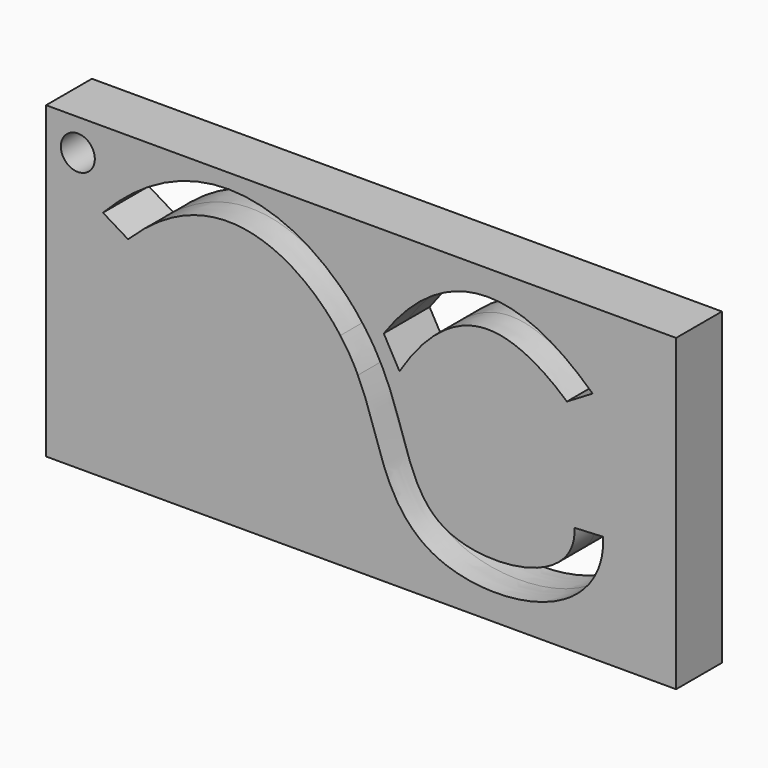
from build123d import *

# Parameters (mm, degrees)
F0_R     = 1.4820473609
F1_DEPTH = 2.5


# Not quite as in the source:
# - ends of sketch curves that miss each other by under 0.0002 mm in the source are joined
# - the dataset's text gives a spline's control points without its knots; the knots are read off the source's solid


with BuildPart() as f1:
    # F0 (on Front) → F1 (new body, symmetric)
    with BuildSketch(Plane.XZ):
        Polygon((0, 8), (0, 35), (-13.424108796, 35), (-19.3373572554, 35), (-55, 35), (-55, 10.4823449254), (-55, 8), align=None)
        with BuildLine():
            add(Edge.make_bspline(
                [(-50.0350917202, 28.3529292792), (-41.4125684769, 37.3503428815), (-32.6083595452, 33.5266259227), (-27.9510231414, 27.9673930825)],
                knots=[0, 0, 0, 0, 0.3600130252, 0.3600130252, 0.3600130252, 0.3600130252], degree=3))
            add(Edge.make_bspline(
                [(-27.9510231414, 27.9673930825), (-27.3487030898, 27.2484333336), (-26.8157416051, 26.5004461928), (-26.3615016308, 25.7474105413)],
                knots=[0.3600130252, 0.3600130252, 0.3600130252, 0.3600130252, 0.4065724843, 0.4065724843, 0.4065724843, 0.4065724843], degree=3))
            add(Edge.make_bspline(
                [(-26.3615016308, 25.7474105413), (-23.3397086824, 20.7379046624), (-24.2248666361, 10.7119674387), (-8.6427712057, 12.8800264919), (-8.8683726817, 17.5248406146)],
                knots=[0.4065724843, 0.4065724843, 0.4065724843, 0.4065724843, 0.7163053419, 1, 1, 1, 1], degree=3))
            Line((-8.8683726817, 17.5248406146), (-6.3713163551, 17.6461241747))
            add(Edge.make_bspline(
                [(-27.7799857666, 23.1064623069), (-27.5788263546, 22.6828182601), (-27.2052833118, 21.8051538248), (-26.5538623577, 19.9878085153), (-25.9771348931, 18.1048414361), (-25.261157142, 16.2105369006), (-24.5732041008, 14.7953607109), (-23.6380951501, 13.4207286348), (-22.5790746848, 12.3877665289), (-21.564555015, 11.6972592795), (-20.7224373548, 11.2571965743), (-19.8357740563, 10.9114121519), (-18.6155851221, 10.5608139887), (-17.024910383, 10.3056128104), (-15.0584946055, 10.2646454513), (-13.0865401909, 10.492714956), (-11.1638473783, 11.0168183507), (-9.6484283114, 11.7525836632), (-8.5378543638, 12.580223758), (-7.781569025, 13.3385124482), (-7.1393061965, 14.2447169704), (-6.6593512732, 15.2903158401), (-6.3849771302, 16.4401002198), (-6.3517175883, 17.2426133896), (-6.3713163551, 17.6461241747)],
                knots=[0.4388333181, 0.4388333181, 0.4388333181, 0.4388333181, 0.46875, 0.5, 0.5625, 0.59375, 0.625, 0.65625, 0.6875, 0.703125, 0.71875, 0.734375, 0.75, 0.78125, 0.8125, 0.84375, 0.875, 0.90625, 0.921875, 0.9375, 0.953125, 0.96875, 0.984375, 1, 1, 1, 1], degree=3))
            add(Edge.make_bspline(
                [(-29.3100691332, 25.6568229932), (-29.175893814, 25.4766680673), (-28.8945520273, 25.081058775), (-28.5026126507, 24.4697850699), (-28.1349969346, 23.8229909625), (-27.9034448496, 23.3653444059), (-27.7889509819, 23.1253431538), (-27.7799857666, 23.1064623069)],
                knots=[0.3774181382, 0.3774181382, 0.3774181382, 0.3774181382, 0.390625, 0.40625, 0.421875, 0.4375, 0.4388333181, 0.4388333181, 0.4388333181, 0.4388333181], degree=3))
            add(Edge.make_bspline(
                [(-47.8384598127, 27.0220131494), (-46.6238688702, 28.2285190868), (-44.7876932656, 29.6157244059), (-42.4668675866, 30.6846781436), (-40.7284615762, 31.1431332011), (-39.0640314859, 31.276428493), (-37.4540401325, 31.1251354681), (-35.8908216692, 30.7151649499), (-33.8798974431, 29.854230091), (-32.0180305429, 28.5725811639), (-30.4090118206, 27.0178615308), (-29.6791632781, 26.1485815571), (-29.3346362458, 25.6898088386), (-29.3100691332, 25.6568229932)],
                knots=[0.0060505396, 0.0060505396, 0.0060505396, 0.0060505396, 0.0625, 0.09375, 0.125, 0.15625, 0.1875, 0.21875, 0.25, 0.3125, 0.34375, 0.375, 0.3774181382, 0.3774181382, 0.3774181382, 0.3774181382], degree=3))
            Line((-47.8384598127, 27.0220131494), (-50.0350917202, 28.3529292792))
        make_face(mode=Mode.SUBTRACT)
        with Locations((-52.2252842784, 32.250855118)):
            Circle(F0_R, mode=Mode.SUBTRACT)
        with BuildLine():
            Line((-24.1447698904, 24.5811181712), (-25.5211698706, 27.0438124237))
            add(Edge.make_bspline(
                [(-25.5211698706, 27.0438124237), (-21.7307303125, 32.4850606553), (-15.5760766078, 36.1038065361), (-7.286220789, 28.3529292792)],
                knots=[0.6763994252, 0.6763994252, 0.6763994252, 0.6763994252, 1, 1, 1, 1], degree=3))
            Line((-7.286220789, 28.3529292792), (-9.5302933464, 27.0140999376))
            add(Edge.make_bspline(
                [(-24.1447698904, 24.5811181712), (-24.1224446589, 24.6175281241), (-23.7978250946, 25.1441069224), (-23.1329260802, 26.1269073446), (-22.0815851014, 27.4069965379), (-20.9608395796, 28.4939738121), (-19.7945426008, 29.3473905624), (-18.6035871508, 29.9436207576), (-17.386494831, 30.2792225731), (-16.0970862388, 30.3511561002), (-14.6559671561, 30.1170615604), (-13.0018113542, 29.4861100301), (-11.2751207696, 28.448266229), (-10.0671772116, 27.4869672564), (-9.5302933464, 27.0140999376)],
                knots=[0.6539337486, 0.6539337486, 0.6539337486, 0.6539337486, 0.65625, 0.6875, 0.71875, 0.75, 0.78125, 0.8125, 0.84375, 0.875, 0.90625, 0.9375, 0.96875, 0.9922543648, 0.9922543648, 0.9922543648, 0.9922543648], degree=3))
        make_face(mode=Mode.SUBTRACT)
    extrude(amount=F1_DEPTH, both=True)


solid = f1.part
